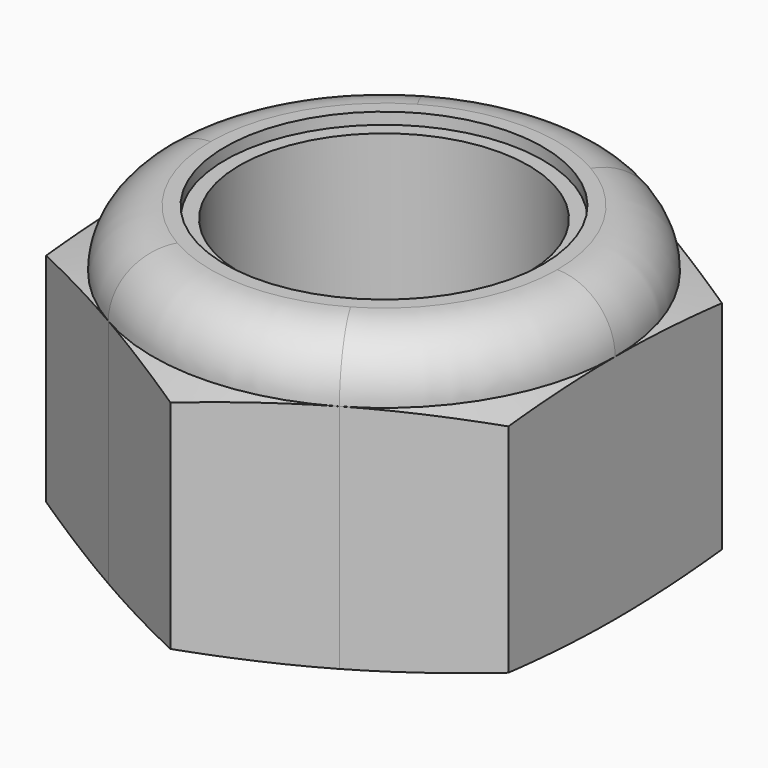
from build123d import *

# Parameters (mm, degrees)
F0_R       = 6
F1_DEPTH   = 4
F2_SIZE2   = 0.4
F2_SIZE    = 2
F2_2_SIZE2 = 0.4
F2_2_SIZE  = 2
F4_DEPTH   = 25
F6_DEPTH   = 1
F7_R       = 0.99999
F8_R       = 2.75
F9_DEPTH   = 0.2
F10_R      = 2.5
F11_DEPTH  = 25


# Not quite as in the source:
# - a fillet or chamfer is up to 0.001 mm smaller than in the source, because OpenCascade refuses the exact size


with BuildPart() as f1:
    # F0 (on Top) → F1 (new body)
    with BuildSketch(Plane.XY):
        Circle(F0_R)
    extrude(amount=F1_DEPTH)

    # F2
    f2_edges = [f1.edges().sort_by_distance(p)[0] for p in [
        (-6, 0, 4),
    ]]
    f2_side = f1.faces().sort_by_distance((0, 0, 4))[0]
    chamfer(f2_edges, length=F2_SIZE, length2=F2_SIZE2, reference=f2_side)

    # F2#2
    f2_2_edges = [f1.edges().sort_by_distance(p)[0] for p in [
        (-6, 0, 0),
    ]]
    f2_2_side = f1.faces().sort_by_distance((0, 0, 0))[0]
    chamfer(f2_2_edges, length=F2_2_SIZE, length2=F2_2_SIZE2, reference=f2_2_side)

    # F3 (on face) → F4 (intersect)
    with BuildSketch(Plane.XY.offset(4)):
        with BuildLine():
            Line((-4, -2.3094010768), (-1.9999999977, -3.4641016165))
            ThreePointArc((-1.9999999977, -3.4641016165), (-3.4641016145, -2.0000000012), (-4, 0))
            Line((-4, 0), (-4, -2.3094010768))
        make_face()
        with BuildLine():
            ThreePointArc((-4, 0), (-3.4641016358, 1.9999999642), (-2.0000000715, 3.4641015738))
            Line((-2.0000000715, 3.4641015738), (-4, 2.3094010768))
            Line((-4, 2.3094010768), (-4, 0))
        make_face()
        with BuildLine():
            ThreePointArc((-2.0000000715, 3.4641015738), (-2.18e-08, 4), (2.0000000338, 3.4641015956))
            Line((2.0000000338, 3.4641015956), (0, 4.6188021535))
            Line((0, 4.6188021535), (-2.0000000715, 3.4641015738))
        make_face()
        with BuildLine():
            Line((4, 0), (4, 2.3094010768))
            Line((4, 2.3094010768), (2.0000000338, 3.4641015956))
            ThreePointArc((2.0000000338, 3.4641015956), (3.4641016249, 1.9999999831), (4, 0))
        make_face()
        with BuildLine():
            Line((4, -2.3094010768), (4, 0))
            ThreePointArc((4, 0), (3.4641016169, -1.9999999969), (2.0000000062, -3.4641016116))
            Line((2.0000000062, -3.4641016116), (4, -2.3094010768))
        make_face()
        with BuildLine():
            Line((0, -4.6188021535), (2.0000000062, -3.4641016116))
            ThreePointArc((2.0000000062, -3.4641016116), (4.9e-09, -4), (-1.9999999977, -3.4641016165))
            Line((-1.9999999977, -3.4641016165), (0, -4.6188021535))
        make_face()
        with BuildLine():
            ThreePointArc((2.0000000062, -3.4641016116), (3.4641016169, -1.9999999969), (4, 0))
            ThreePointArc((4, 0), (3.4641016249, 1.9999999831), (2.0000000338, 3.4641015956))
            ThreePointArc((2.0000000338, 3.4641015956), (-2.18e-08, 4), (-2.0000000715, 3.4641015738))
            ThreePointArc((-2.0000000715, 3.4641015738), (-3.4641016358, 1.9999999642), (-4, 0))
            ThreePointArc((-4, 0), (-3.4641016145, -2.0000000012), (-1.9999999977, -3.4641016165))
            ThreePointArc((-1.9999999977, -3.4641016165), (4.9e-09, -4), (2.0000000062, -3.4641016116))
        make_face()
    extrude(amount=-F4_DEPTH, mode=Mode.INTERSECT)

    # F5 (on face) → F6 (join)
    with BuildSketch(Plane.XY.offset(4)):
        with BuildLine():
            ThreePointArc((1.9999999952, -3.4641016179), (3.4641016138, -2.0000000024), (4, 0))
            ThreePointArc((4, 0), (3.4641016188, 1.9999999936), (2.0000000128, 3.4641016077))
            ThreePointArc((2.0000000128, 3.4641016077), (0, 4), (-2.0000000128, 3.4641016077))
            ThreePointArc((-2.0000000128, 3.4641016077), (-3.4641016188, 1.9999999936), (-4, 0))
            ThreePointArc((-4, 0), (-3.4641016204, -1.9999999909), (-2.0000000181, -3.4641016047))
            ThreePointArc((-2.0000000181, -3.4641016047), (-1.32e-08, -4), (1.9999999952, -3.4641016179))
        make_face()
    extrude(amount=F6_DEPTH)

    # F7 (radius 1 in the source; OpenCascade refuses exactly that, so slightly less here)
    f7_edges = [f1.edges().sort_by_distance(p)[0] for p in [
        (-4, 0, 5),
    ]]
    fillet(f7_edges, radius=F7_R)

    # F8 (on face) → F9 (cut)
    with BuildSketch(Plane.XY.offset(5)):
        Circle(F8_R)
    extrude(amount=-F9_DEPTH, mode=Mode.SUBTRACT)

    # F10 (on face) → F11 (cut)
    with BuildSketch(Plane.XY.offset(4.8)):
        Circle(F10_R)
    extrude(amount=-F11_DEPTH, mode=Mode.SUBTRACT)


solid = f1.part
